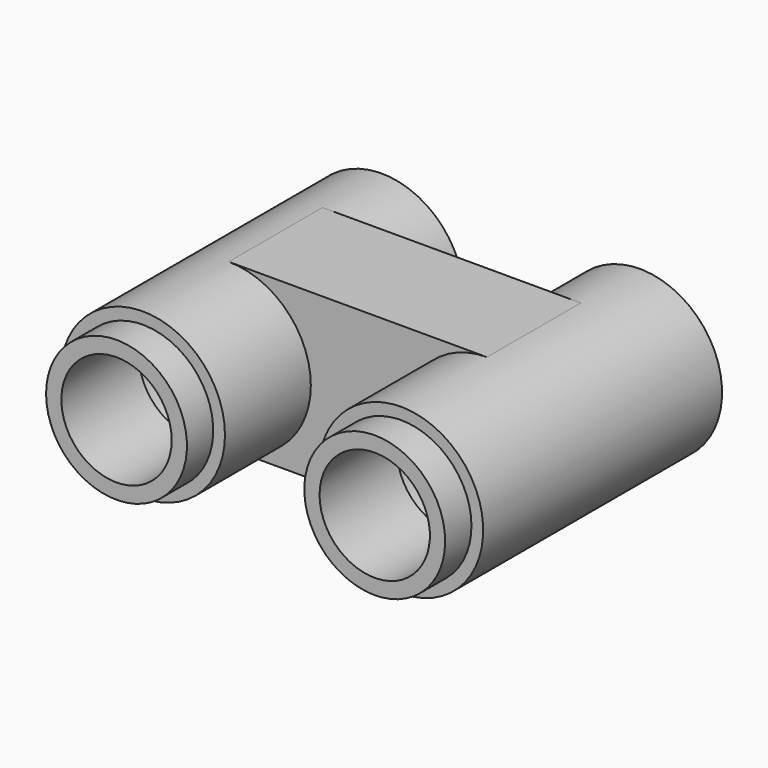
from build123d import *

# Parameters (mm, degrees)
F1_R           = 8.89
F1_R_2         = 5.969
F3_DEPTH       = 3.556
F5_R           = 8.89
F5_R_2         = 7.62
F7_DEPTH       = 3.556
F8_DEPTH       = 25.4
F8_DEPTH_BACK  = 25.4
F0_W           = 10.282781499
F0_H           = 12.7
F0_W_2         = 17.657218501
F11_DEPTH      = 8.89
F11_DEPTH_BACK = 8.89
F9_R           = 7.62
F10_R          = 7.62
F12_DEPTH      = 25.4


# Not quite as in the source:
# - a feature of the source that left no trace in its solid (it failed there, or was rolled back) is left out
# - a pattern or mirror of a feature is missing from the dataset's text; its kind, count and spacing are read off the source's solid


with BuildPart() as f2:
    # F2: sweep along a path in F0
    with BuildLine(Plane.XY) as f2_path:
        Line((0, 0), (0, 70.4088))
        ThreePointArc((0, 70.4088), (13.97, 84.3788), (27.94, 70.4088))
        Line((27.94, 70.4088), (27.94, 0))
        Line((27.94, 0), (27.94, -3.556))
    # F1 (on Front) → F2 (sweep)
    with BuildSketch(Plane.XZ):
        Circle(F1_R)
        Circle(F1_R_2, mode=Mode.SUBTRACT)
    sweep(path=f2_path.line)

    # F3 (add): a face of the model
    f3_faces = [f2.faces().sort_by_distance(p)[0] for p in [
        (-8.6385528286, 0, 0),
    ]]
    extrude(f3_faces, amount=F3_DEPTH)

    # F5 (on face) → F7 (cut)
    with BuildSketch(Plane.XZ.offset(3.556)):
        with Locations((27.94, 0)):
            Circle(F5_R)
        with Locations((27.94, 0)):
            Circle(F5_R_2, mode=Mode.SUBTRACT)
    f7 = extrude(amount=-F7_DEPTH, mode=Mode.SUBTRACT)

    # F7_copies: F7 across plane
    add(f7.mirror(Plane(origin=(13.97, 0, 0), x_dir=(0, 0, -1), z_dir=(-1, 0, 0))), mode=Mode.SUBTRACT)

    # F0 (on Top) → F8 (cut, two sides)
    with BuildSketch(Plane.XY) as f8_sk:
        with BuildLine():
            Line((-21.5208670124, 32.3088), (0, 32.3088))
            Line((0, 32.3088), (0, 70.4088))
            ThreePointArc((0, 70.4088), (13.97, 84.3788), (27.94, 70.4088))
            Line((27.94, 70.4088), (27.94, 32.3088))
            Line((27.94, 32.3088), (57.1982562542, 32.3088))
            Line((57.1982562542, 32.3088), (57.1982562542, 105.6616994024))
            Line((57.1982562542, 105.6616994024), (-21.5208670124, 105.6616994024))
            Line((-21.5208670124, 105.6616994024), (-21.5208670124, 32.3088))
        make_face()
        with BuildLine():
            Line((0, 70.4088), (0, 32.3088))
            Line((0, 32.3088), (13.97, 32.3088))
            Line((13.97, 32.3088), (27.94, 32.3088))
            Line((27.94, 32.3088), (27.94, 70.4088))
            ThreePointArc((27.94, 70.4088), (13.97, 84.3788), (0, 70.4088))
        make_face()
    extrude(amount=-F8_DEPTH, mode=Mode.SUBTRACT)
    extrude(f8_sk.sketch, amount=F8_DEPTH_BACK, mode=Mode.SUBTRACT)

    # F0 (on Top) → F11 (join, two sides)
    with BuildSketch(Plane.XY) as f11_sk:
        with Locations((22.7986092505, 17.9638495505)):
            Rectangle(F0_W, F0_H)
        with Locations((8.8286092505, 17.9638495505)):
            Rectangle(F0_W_2, F0_H)
    extrude(amount=F11_DEPTH)
    extrude(f11_sk.sketch, amount=-F11_DEPTH_BACK)

    # F9 (on face) + F10 (on face) → F12 (cut)
    with BuildSketch(Plane(origin=(0, 32.3088, 0), x_dir=(-1, 0, 0), z_dir=(0, 1, 0))):
        with Locations((-27.94, 0)):
            Circle(F9_R)
    with BuildSketch(Plane(origin=(0, 32.3088, 0), x_dir=(-1, 0, 0), z_dir=(0, 1, 0))):
        Circle(F10_R)
    extrude(amount=-F12_DEPTH, mode=Mode.SUBTRACT)


solid = f2.part
